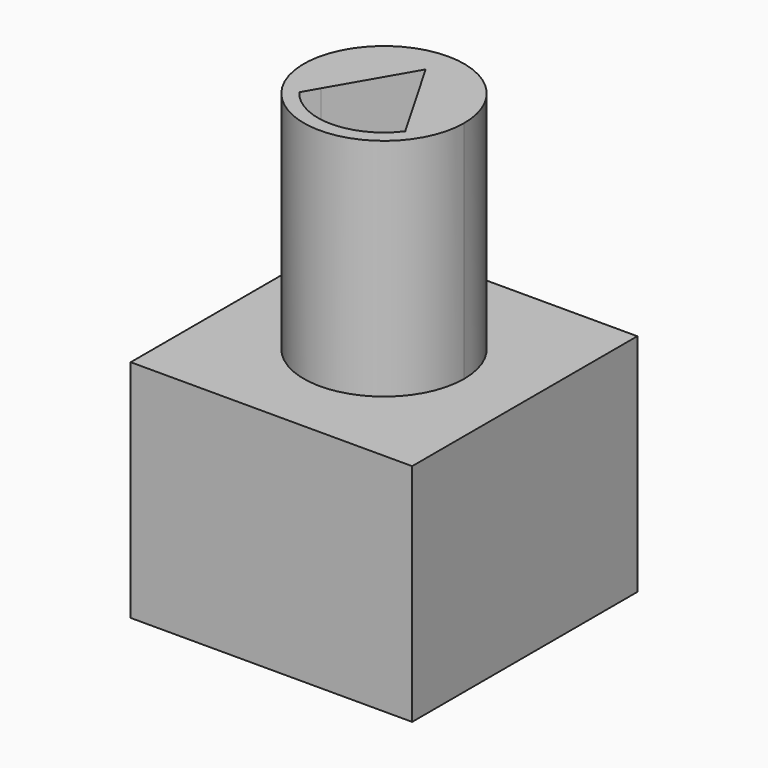
from build123d import *

# Parameters (mm, degrees)
F1_DEPTH = 8
F2_DEPTH = 3
F3_W     = 10
F3_H     = 10
F4_DEPTH = 8


with BuildPart() as f1:
    # F0 (on Top) → F1 (new body)
    with BuildSketch(Plane.XY):
        with BuildLine():
            ThreePointArc((0, 2.85), (-2.0152543264, -2.0152543264), (2.85, 0))
            ThreePointArc((2.85, 0), (2.0152543264, 2.0152543264), (0, 2.85))
        make_face()
        with BuildLine():
            ThreePointArc((-1.8812210579, -1.4083704525), (-2.1014483771, 1.0518624997), (0, 2.35))
            ThreePointArc((0, 2.35), (1.6617009358, 1.6617009358), (2.35, 0))
            ThreePointArc((2.35, 0), (2.2297275042, -0.7421692913), (1.8812210579, -1.4083704525))
            ThreePointArc((1.8812210579, -1.4083704525), (0, -2.35), (-1.8812210579, -1.4083704525))
        make_face(mode=Mode.SUBTRACT)
        with BuildLine():
            ThreePointArc((2.35, 0), (1.6617009358, 1.6617009358), (0, 2.35))
            Line((0, 2.35), (0, 1.85))
            Line((0, 1.85), (1.5588457268, -0.85))
            Line((1.5588457268, -0.85), (1.8812210579, -1.4083704525))
            ThreePointArc((1.8812210579, -1.4083704525), (2.2297275042, -0.7421692913), (2.35, 0))
        make_face()
        with BuildLine():
            Line((0, 1.85), (0, 2.35))
            ThreePointArc((0, 2.35), (-2.1014483771, 1.0518624997), (-1.8812210579, -1.4083704525))
            Line((-1.8812210579, -1.4083704525), (-1.5588457268, -0.85))
            Line((-1.5588457268, -0.85), (0, 1.85))
        make_face()
    extrude(amount=F1_DEPTH)

    # F0 (on Top) → F2 (join)
    with BuildSketch(Plane.XY):
        with BuildLine():
            Line((-1.5588457268, -0.85), (-1.8812210579, -1.4083704525))
            ThreePointArc((-1.8812210579, -1.4083704525), (0, -2.35), (1.8812210579, -1.4083704525))
            Line((1.8812210579, -1.4083704525), (1.5588457268, -0.85))
            Line((1.5588457268, -0.85), (0, 1.85))
            Line((0, 1.85), (-1.5588457268, -0.85))
        make_face()
    extrude(amount=F2_DEPTH)

    # F3 (on Top) → F4 (join)
    with BuildSketch(Plane.XY):
        Rectangle(F3_W, F3_H)
    extrude(amount=-F4_DEPTH)


solid = f1.part
